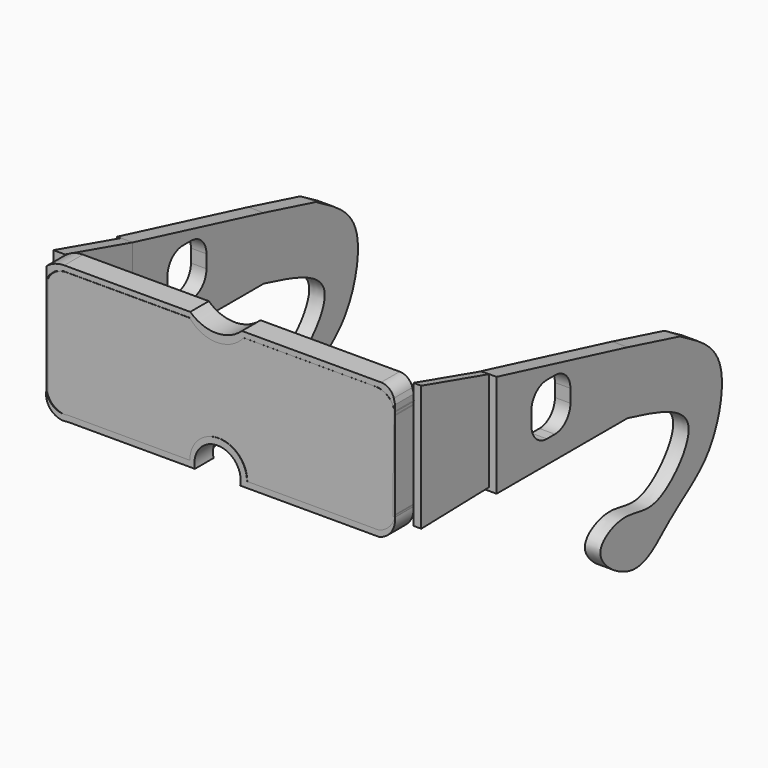
from build123d import *

# Parameters (mm, degrees)
F1_DEPTH  = 7.62
F5_DEPTH  = 2.54
F7_DEPTH  = 0.0254
F9_DEPTH  = 3.81
F11_DEPTH = 2.54
F12_DEPTH = 5.08
F13_DEPTH = 5.08
F15_DEPTH = 1.778
F17_DEPTH = 25.4
F19_DEPTH = 25.4
F21_DEPTH = 86.3034930606
F23_DEPTH = 7.62
F25_DEPTH = 7.62
F27_DEPTH = 7.62
F29_DEPTH = 7.62


# Not quite as in the source:
# - the dataset's text gives a spline's control points without its knots; the knots are read off the source's solid


with BuildPart() as f1:
    # F0 (on Front) → F1 (new body)
    with BuildSketch(Plane.XZ):
        with BuildLine():
            ThreePointArc((-49.7503069009, 27.6395086206), (-54.2404349615, 25.7796366811), (-56.1003069009, 21.2895086206))
            Line((-56.1003069009, 21.2895086206), (-56.1003069009, 0))
            Line((-56.1003069009, 0), (-56.1003069009, -7.2984495926))
            ThreePointArc((-56.1003069009, -7.2984495926), (-54.2404349615, -11.7885776531), (-49.7503069009, -13.6484495926))
            Line((-49.7503069009, -13.6484495926), (-9.0169999748, -13.6484495926))
            ThreePointArc((-9.0169999748, -13.6484495926), (0.38100034, -3.971437742), (9.7790006548, -13.6484495926))
            Line((9.7790006548, -13.6484495926), (51.8496930991, -13.6484495926))
            ThreePointArc((51.8496930991, -13.6484495926), (56.3398211596, -11.7885776531), (58.1996930991, -7.2984495926))
            Line((58.1996930991, -7.2984495926), (58.1996930991, 21.2895086206))
            ThreePointArc((58.1996930991, 21.2895086206), (56.3398211596, 25.7796366811), (51.8496930991, 27.6395086206))
            Line((51.8496930991, 27.6395086206), (8.5893462526, 27.6395086206))
            ThreePointArc((8.5893462526, 27.6395086206), (-0.2138268611, 23.5515440161), (-9.0169999748, 27.6395086206))
            Line((-9.0169999748, 27.6395086206), (-49.7503069009, 27.6395086206))
        make_face()
    extrude(amount=F1_DEPTH)

    # F20 (on face) → F21 (cut, through all)
    with BuildSketch(Plane.XY.offset(27.6395086206)):
        with BuildLine():
            Line((57.1385622025, 0), (-55.5774010718, 0))
            ThreePointArc((-55.5774010718, 0), (0.7805805653, -3.8925180506), (57.1385622025, 0))
        make_face()
    extrude(amount=-F21_DEPTH, mode=Mode.SUBTRACT)


with BuildPart() as f5:
    # F4 (on face) → F5 (new body)
    with BuildSketch(Plane(origin=(0, 0, 0), x_dir=(-1, 0, 0), z_dir=(0, 1, 0))):
        with BuildLine():
            add(Edge.make_bspline(
                [(-12.4614257365, -13.6484495926), (-12.1586115866, -10.4173610488), (-11.5280396934, -3.6890307499), (0.0066860275, 2.099838112), (11.3074356161, -4.3078050469), (11.1437820154, -10.6614531988), (11.0668446869, -13.6484495926)],
                knots=[0, 0, 0, 0, 0.2426529219, 0.5052937994, 0.7674272163, 1, 1, 1, 1], degree=3))
            Line((-12.4614257365, -13.6484495926), (-9.7790006548, -13.6484495926))
            ThreePointArc((-9.7790006548, -13.6484495926), (-0.38100034, -3.9068475717), (9.0169999748, -13.6484495926))
            Line((9.0169999748, -13.6484495926), (11.0668446869, -13.6484495926))
        make_face()
    extrude(amount=F5_DEPTH)


with BuildPart() as f7:
    # F6 (on face) → F7 (new body)
    with BuildSketch(Plane(origin=(0, 0, 0), x_dir=(-1, 0, 0), z_dir=(0, 1, 0))):
        with BuildLine():
            Line((42.3234785444, -11.7885776531), (50.8534041696, -11.7885776531))
            ThreePointArc((50.8534041696, -11.7885776531), (51.4686118723, -11.533750279), (51.7234392464, -10.9185425763))
            Line((51.7234392464, -10.9185425763), (51.7234392464, -5.4207351527))
            ThreePointArc((51.7234392464, -5.4207351527), (51.4686118723, -4.8055274501), (50.8534041696, -4.5507000759))
            Line((50.8534041696, -4.5507000759), (42.3234785444, -4.5507000759))
            ThreePointArc((42.3234785444, -4.5507000759), (41.7082708417, -4.8055274501), (41.4534434676, -5.4207351527))
            Line((41.4534434676, -5.4207351527), (41.4534434676, -10.9185425763))
            ThreePointArc((41.4534434676, -10.9185425763), (41.7082708417, -11.533750279), (42.3234785444, -11.7885776531))
        make_face()
    extrude(amount=F7_DEPTH)


with BuildPart() as f7b:
    # F6 (on face) → F7, piece 2 (new body)
    with BuildSketch(Plane(origin=(0, 0, 0), x_dir=(-1, 0, 0), z_dir=(0, 1, 0))):
        with BuildLine():
            ThreePointArc((-53.392957896, -10.9185425763), (-53.1381305219, -11.533750279), (-52.5229228192, -11.7885776531))
            Line((-52.5229228192, -11.7885776531), (-43.9930009193, -11.7885776531))
            ThreePointArc((-43.9930009193, -11.7885776531), (-43.3777932166, -11.533750279), (-43.1229658425, -10.9185425763))
            Line((-43.1229658425, -10.9185425763), (-43.1229658425, -5.4207351527))
            ThreePointArc((-43.1229658425, -5.4207351527), (-43.3777932166, -4.8055274501), (-43.9930009193, -4.5507000759))
            Line((-43.9930009193, -4.5507000759), (-52.5229228192, -4.5507000759))
            ThreePointArc((-52.5229228192, -4.5507000759), (-53.1381305219, -4.8055274501), (-53.392957896, -5.4207351527))
            Line((-53.392957896, -5.4207351527), (-53.392957896, -10.9185425763))
        make_face()
    extrude(amount=F7_DEPTH)


with BuildPart() as f9:
    # F8 (on face) → F9 (new body)
    with BuildSketch(Plane(origin=(-56.1003069009, 0, 0), x_dir=(0, -1, 0), z_dir=(-1, 0, 0))):
        Polygon((0, 21.2895086206), (0, 27.5897663087), (-27.7157612145, 19.8064111173), (-27.7157612145, -12.5891771168), (0, -14.061704278), (0, -7.2984495926), align=None)
    extrude(amount=F9_DEPTH)


with BuildPart() as f11:
    # F10 (on face) → F11 (new body)
    with BuildSketch(Plane.YZ.offset(58.1996930991)):
        Polygon((27.795067057, 19.716065377), (0, 27.6761949062), (0, -13.6280357838), (27.795067057, -12.9204681143), align=None)
    extrude(amount=F11_DEPTH)


with BuildPart() as f12:
    # F2 (on face) → F12 (new body)
    with BuildSketch(Plane(origin=(-56.1003069009, 0, 0), x_dir=(0, -1, 0), z_dir=(-1, 0, 0))):
        with BuildLine():
            Line((-27.7196131647, 19.7965819389), (-81.4566115099, 6.5045165328))
            Line((-81.4566115099, 6.5045165328), (-102.8235959408, 0.9310996321))
            add(Edge.make_bspline(
                [(-102.8235959408, 0.9310996321), (-107.8599103248, -1.872827049), (-117.2462147867, -7.0985749892), (-121.7922997723, -19.5676011266), (-115.8589131877, -40.0486212115), (-98.685173686, -48.8287854459), (-85.877858555, -63.9450201534), (-63.9998710118, -48.0559280032), (-80.8552011489, -39.6724741723), (-93.3752134157, -47.4141506036), (-115.9475150956, -22.642313665), (-93.5251936786, -16.9969477572), (-81.4566115099, -13.9583880531)],
                knots=[0, 0, 0, 0, 0.0967317031, 0.1802812825, 0.286237306, 0.3922544833, 0.4923884516, 0.5923909155, 0.6731656718, 0.7629520201, 0.8724113811, 1, 1, 1, 1], degree=3))
            Line((-81.4566115099, -13.9583880531), (-27.7196131647, -13.9583880531))
            Line((-27.7196131647, -13.9583880531), (-27.7196131647, 19.7965819389))
        make_face()
    extrude(amount=F12_DEPTH)

    # F16 (on face) → F17 (cut)
    with BuildSketch(Plane(origin=(-61.1803069009, 0, 0), x_dir=(0, -1, 0), z_dir=(-1, 0, 0))):
        with BuildLine():
            Line((-41.9807806611, -0.1296451479), (-41.9807806611, 4.1883554474))
            ThreePointArc((-41.9807806611, 4.1883554474), (-43.8406526006, 8.6784835079), (-48.3307806611, 10.5383554474))
            Line((-48.3307806611, 10.5383554474), (-51.6327800393, 10.5383554474))
            ThreePointArc((-51.6327800393, 10.5383554474), (-56.1229080998, 8.6784835079), (-57.9827800393, 4.1883554474))
            Line((-57.9827800393, 4.1883554474), (-57.9827800393, -0.1296451479))
            ThreePointArc((-57.9827800393, -0.1296451479), (-56.1229080998, -4.6197732085), (-51.6327800393, -6.4796451479))
            Line((-51.6327800393, -6.4796451479), (-48.3307806611, -6.4796451479))
            ThreePointArc((-48.3307806611, -6.4796451479), (-43.8406526006, -4.6197732085), (-41.9807806611, -0.1296451479))
        make_face()
    extrude(amount=-F17_DEPTH, mode=Mode.SUBTRACT)


with BuildPart() as f13:
    # F3 (on face) → F13 (new body)
    with BuildSketch(Plane.YZ.offset(58.1996930991)):
        with BuildLine():
            Line((102.8235959408, 0.9310996321), (81.4566115099, 6.5045165328))
            Line((81.4566115099, 6.5045165328), (27.7196131647, 19.7965819389))
            Line((27.7196131647, 19.7965819389), (27.7196131647, -13.9583880531))
            Line((27.7196131647, -13.9583880531), (81.4566115099, -13.9583880531))
            add(Edge.make_bspline(
                [(102.8235959408, 0.9310996321), (107.8599103248, -1.872827049), (117.2462147867, -7.0985749892), (121.7922997723, -19.5676011266), (115.8589131877, -40.0486212115), (98.685173686, -48.8287854459), (85.877858555, -63.9450201534), (63.9998710118, -48.0559280032), (80.8552011489, -39.6724741723), (93.3752134157, -47.4141506036), (115.9475150956, -22.642313665), (93.5251936786, -16.9969477572), (81.4566115099, -13.9583880531)],
                knots=[0, 0, 0, 0, 0.0967317031, 0.1802812825, 0.286237306, 0.3922544833, 0.4923884516, 0.5923909155, 0.6731656718, 0.7629520201, 0.8724113811, 1, 1, 1, 1], degree=3))
        make_face()
    extrude(amount=F13_DEPTH)

    # F18 (on face) → F19 (cut)
    with BuildSketch(Plane.YZ.offset(63.2796930991)):
        with BuildLine():
            ThreePointArc((48.3307806611, 10.5383554474), (43.8406526006, 8.6784835079), (41.9807806611, 4.1883554474))
            Line((41.9807806611, 4.1883554474), (41.9807806611, -0.1296451479))
            ThreePointArc((41.9807806611, -0.1296451479), (43.8406526006, -4.6197732085), (48.3307806611, -6.4796451479))
            Line((48.3307806611, -6.4796451479), (51.6327800393, -6.4796451479))
            ThreePointArc((51.6327800393, -6.4796451479), (56.1229080998, -4.6197732085), (57.9827800393, -0.1296451479))
            Line((57.9827800393, -0.1296451479), (57.9827800393, 4.1883554474))
            ThreePointArc((57.9827800393, 4.1883554474), (56.1229080998, 8.6784835079), (51.6327800393, 10.5383554474))
            Line((51.6327800393, 10.5383554474), (48.3307806611, 10.5383554474))
        make_face()
    extrude(amount=-F19_DEPTH, mode=Mode.SUBTRACT)


with BuildPart() as f15:
    # F14 (on face) → F15 (new body)
    with BuildSketch(Plane(origin=(0, 0, 0), x_dir=(-1, 0, 0), z_dir=(0, 1, 0))):
        with BuildLine():
            Line((-8.7629994377, 25.9053539485), (-52.9589988291, 25.9053539485))
            add(Edge.make_bspline(
                [(-52.9589988291, 25.9053539485), (-53.75376482, 26.025301797), (-55.2776016348, 26.2552826334), (-56.408415892, 24.4881555365), (-57.0703809138, 21.5426962408), (-56.9225391452, 20.1348025884), (-56.8558573723, 19.4997936487)],
                knots=[0, 0, 0, 0, 0.245570954, 0.4708430716, 0.7613318453, 1, 1, 1, 1], degree=3))
            Line((-56.8558573723, 19.4997936487), (-54.6920225024, 19.4997936487))
            add(Edge.make_bspline(
                [(-54.6920225024, 19.4997936487), (-54.9611840238, 21.260593036), (-55.405370764, 24.1663714548), (-53.6504854469, 24.0472802428), (-52.9589988291, 24.0003541112)],
                knots=[0, 0, 0, 0, 0.6059647824, 1, 1, 1, 1], degree=3))
            Line((-52.9589988291, 24.0003541112), (-8.7629994377, 24.0003541112))
            ThreePointArc((-8.7629994377, 24.0003541112), (0.1270002685, 21.1256435044), (9.0169999748, 24.0003541112))
            Line((9.0169999748, 24.0003541112), (52.4509996176, 24.0003541112))
            add(Edge.make_bspline(
                [(52.4509996176, 25.9053539485), (52.9636924518, 25.6153477978), (54.0337816476, 25.01004882), (55.4813546233, 23.7236023347), (56.1804331848, 17.7616535207), (53.036677573, 18.3870579991), (53.6884567777, 20.6552843527), (53.9895347077, 23.257215023), (52.9184158941, 23.7745839564), (52.4509996176, 24.0003541112)],
                knots=[0, 0, 0, 0, 0.1260212173, 0.2630306765, 0.4751276596, 0.5966597822, 0.733288043, 0.8836118755, 1, 1, 1, 1], degree=3))
            Line((52.4509996176, 25.9053539485), (9.0169999748, 25.9053539485))
            ThreePointArc((9.0169999748, 25.9053539485), (0.1270002685, 22.7743020538), (-8.7629994377, 25.9053539485))
        make_face()
    extrude(amount=F15_DEPTH)


with BuildPart() as f23:
    # F22 (on Front) → F23 (new body)
    with BuildSketch(Plane.XZ):
        with BuildLine():
            Line((-8.9364983141, 29.4457860291), (-50.245679915, 29.4457860291))
            ThreePointArc((-50.245679915, 29.4457860291), (-53.3525559473, 28.9023832068), (-56.0905449092, 27.3366943002))
            Line((-56.0905449092, 27.3366943002), (-56.0905449092, 22.2639869899))
            add(Edge.make_bspline(
                [(-50.245679915, 27.6848748326), (-50.4285049906, 27.7143390453), (-50.8661484293, 27.7848699574), (-51.8111565891, 27.0645822641), (-53.2460370225, 26.9833890204), (-54.3418045719, 25.7407718325), (-55.5724178579, 24.8306770642), (-55.9023930831, 23.1960507054), (-56.0905449092, 22.2639869899)],
                knots=[0, 0, 0, 0, 0.1071720922, 0.2565466623, 0.4238476079, 0.6010705191, 0.7725304671, 1, 1, 1, 1], degree=3))
            Line((-50.245679915, 27.6848748326), (-9.7019709647, 27.6848748326))
            Line((-9.7019709647, 27.6848748326), (-9.1517250985, 27.6848748326))
            ThreePointArc((-9.1517250985, 27.6848748326), (-0.2824102319, 23.4524670185), (8.6027514189, 27.6515055448))
            Line((8.6027514189, 27.6515055448), (51.0343462229, 27.6515055448))
            add(Edge.make_bspline(
                [(58.2171657118, 22.8821949653), (58.071740031, 23.3127251238), (57.2605463845, 24.5552954967), (56.7492047464, 25.4876571931), (55.7487483013, 26.4116373045), (54.6358184154, 27.002702597), (53.0973639035, 27.6947707232), (51.7484769867, 27.6664821469), (51.0343462229, 27.6515055448)],
                knots=[0.0906408008, 0.0906408008, 0.0906408008, 0.0906408008, 0.2581763529, 0.3900768326, 0.5285148886, 0.6667154201, 0.8235517236, 1, 1, 1, 1], degree=3))
            add(Edge.make_bspline(
                [(58.2726368512, 22.6464999569), (58.2638400685, 22.7167462545), (58.2469886145, 22.7939047887), (58.2171657118, 22.8821949653)],
                knots=[0.0562837571, 0.0562837571, 0.0562837571, 0.0562837571, 0.0906408008, 0.0906408008, 0.0906408008, 0.0906408008], degree=3))
            Line((58.2726368512, 22.6464999569), (58.2726368512, 24.5137837211))
            Line((58.2726368512, 24.5137837211), (57.8246861696, 26.2277424335))
            ThreePointArc((57.8246861696, 26.2277424335), (56.2900496098, 28.5476305929), (53.657501936, 29.4457860291))
            Line((53.657501936, 29.4457860291), (8.0137364566, 29.4457860291))
            ThreePointArc((8.0137364566, 29.4457860291), (-0.4613809288, 26.1084372425), (-8.9364983141, 29.4457860291))
        make_face()
        with BuildLine():
            add(Edge.make_bspline(
                [(58.2726368512, 22.3383679986), (58.279842302, 22.4348951861), (58.2870477528, 22.5314223737), (58.2726368512, 22.6464999569)],
                knots=[0, 0, 0, 0, 0.0562837571, 0.0562837571, 0.0562837571, 0.0562837571], degree=3))
            Line((58.2726368512, 22.6464999569), (58.2726368512, 22.3383679986))
        make_face()
        with BuildLine():
            Line((58.2726368512, 22.3383679986), (58.2726368512, 22.6464999569))
            add(Edge.make_bspline(
                [(58.2726368512, 22.6464999569), (58.2638400685, 22.7167462545), (58.2469886145, 22.7939047887), (58.2171657118, 22.8821949653)],
                knots=[0.0562837571, 0.0562837571, 0.0562837571, 0.0562837571, 0.0906408008, 0.0906408008, 0.0906408008, 0.0906408008], degree=3))
            Line((58.2171657118, 22.8821949653), (58.2726368512, 22.3383679986))
        make_face()
    extrude(amount=F23_DEPTH)


with BuildPart() as f25:
    # F24 (on Front) → F25 (new body)
    with BuildSketch(Plane.XZ):
        Polygon((-56.1131052673, 22.561211139), (-56.1269335449, -8.9126545936), (-55.5592104793, -8.9126545936), (-55.5592104793, 24.3334937841), align=None)
    extrude(amount=F25_DEPTH)


with BuildPart() as f27:
    # F26 (on Front) → F27 (new body)
    with BuildSketch(Plane.XZ):
        Polygon((58.1854842603, -7.9826498404), (58.1854842603, 23.0242200196), (57.873763144, 23.6146841198), (57.5063675642, -7.9826498404), align=None)
    extrude(amount=F27_DEPTH)


with BuildPart() as f29:
    # F28 (on Front) → F29 (new body)
    with BuildSketch(Plane.XZ):
        with BuildLine():
            ThreePointArc((-56.1637729406, -8.9156040922), (-54.3306631075, -14.0125840828), (-49.0927030332, -15.3921749443))
            Line((-49.0927030332, -15.3921749443), (-7.4029914103, -15.3921749443))
            ThreePointArc((-7.4029914103, -15.3921749443), (0.017864164, -6.2133918925), (7.4387197383, -15.3921749443))
            Line((7.4387197383, -15.3921749443), (52.9686175287, -15.3921749443))
            ThreePointArc((52.9686175287, -15.3921749443), (56.9707726689, -12.7209616367), (58.182310313, -8.0642672256))
            ThreePointArc((58.182310313, -8.0642672256), (56.2780660321, -11.4362778272), (52.9686175287, -13.4472856298))
            Line((52.9686175287, -13.4472856298), (9.6552046016, -13.4472856298))
            ThreePointArc((9.6552046016, -13.4472856298), (0.2913875505, -4.0171578928), (-9.0724295005, -13.4472856298))
            Line((-9.0724295005, -13.4472856298), (-49.0927030332, -13.4472856298))
            ThreePointArc((-49.0927030332, -13.4472856298), (-53.5694621765, -12.650096616), (-56.1637729406, -8.9156040922))
        make_face()
    extrude(amount=F29_DEPTH)


solid = Compound([f1.part, f5.part, f7.part, f7b.part, f9.part, f11.part, f12.part, f13.part, f15.part, f23.part, f25.part, f27.part, f29.part])
